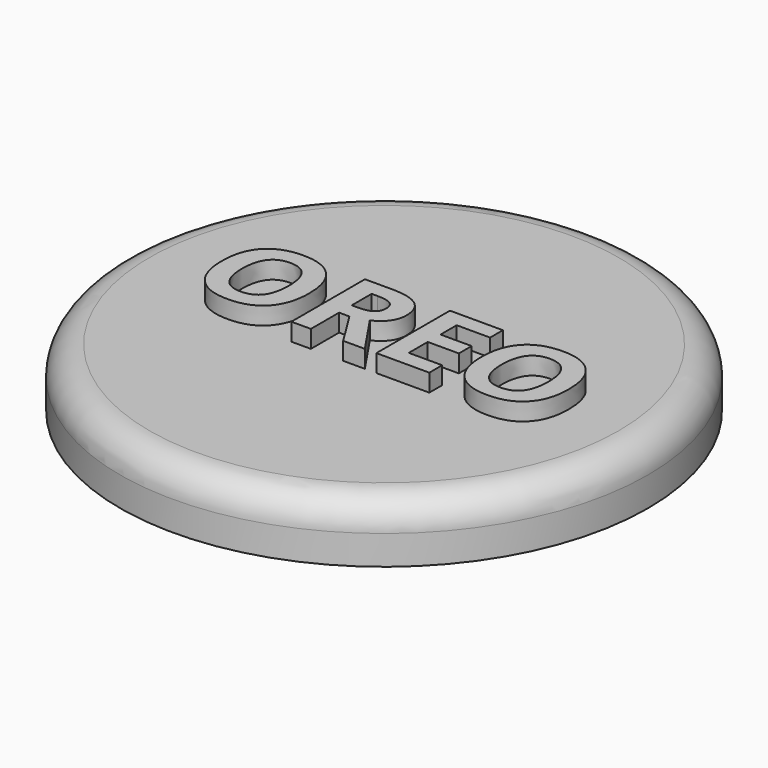
from build123d import *

# Parameters (mm, degrees)
F0_R         = 45
F1_DEPTH     = 10
F2_R         = 5
F3_TEXT_SIZE = 21.9549647429
F4_DEPTH     = 3


# Not quite as in the source:
# - Text() gives the source's letters only with a copy of the font that has no kerning and outlines rounded to 1/6400 em; it was checked with that copy


with BuildPart() as f1:
    # F0 (on Top) → F1 (new body)
    with BuildSketch(Plane.XY):
        Circle(F0_R)
    extrude(amount=-F1_DEPTH)

    # F2
    f2_edges = [f1.edges().sort_by_distance(p)[0] for p in [
        (-45, 0, 0),
    ]]
    fillet(f2_edges, radius=F2_R)

    # F3 (on face) → F4 (join)
    with BuildSketch(Plane.XY):
        with Locations((-29.5273568481, -7.1581481025)):
            Text('OREO', F3_TEXT_SIZE, font='Open Sans', font_style=FontStyle.BOLD, text_align=(TextAlign.LEFT, TextAlign.BOTTOM))
    extrude(amount=F4_DEPTH)


solid = f1.part
